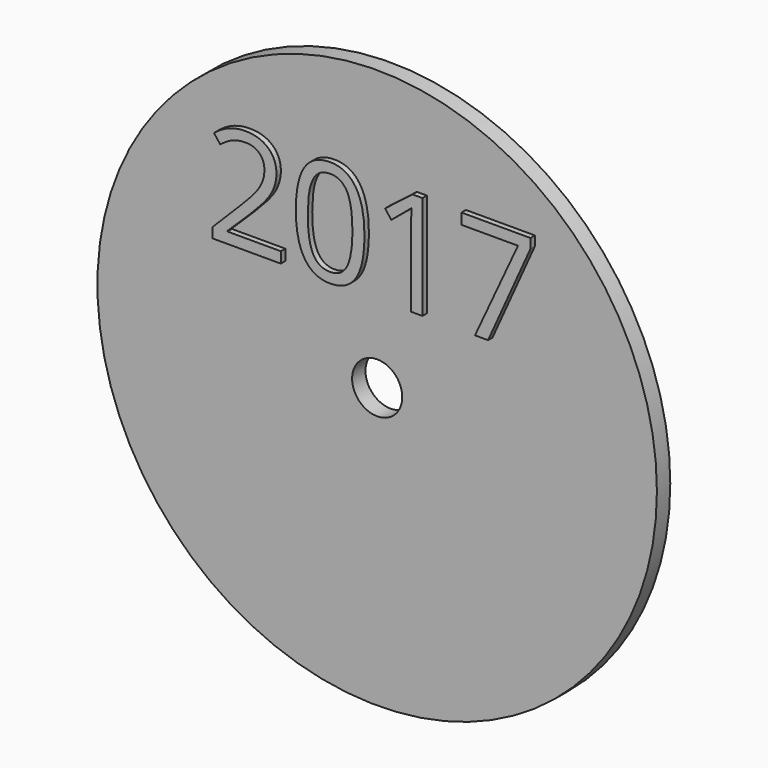
from build123d import *

# Parameters (mm, degrees)
F0_R         = 50.2
F0_R_2       = 4.5
F1_DEPTH     = 3
F4_TEXT_SIZE = 26.0763275839
F5_DEPTH     = 1


# Not quite as in the source:
# - the program builds the solid bodies; features that only make, move or delete a surface that nothing else refers to are left out
# - Text() gives the source's letters only with a copy of the font that has no kerning and outlines rounded to 1/6400 em; it was checked with that copy


with BuildPart() as f1:
    # F0 (on Front) → F1 (new body)
    with BuildSketch(Plane.XZ):
        Circle(F0_R)
        Circle(F0_R_2, mode=Mode.SUBTRACT)
    extrude(amount=F1_DEPTH)

    # F4 (on face) → F5 (join)
    with BuildSketch(Plane.XZ.offset(3)):
        with Locations((-30, 14.664138422)):
            Text('2017', F4_TEXT_SIZE, font='Open Sans', text_align=(TextAlign.LEFT, TextAlign.BOTTOM))
    extrude(amount=F5_DEPTH)


solid = f1.part
